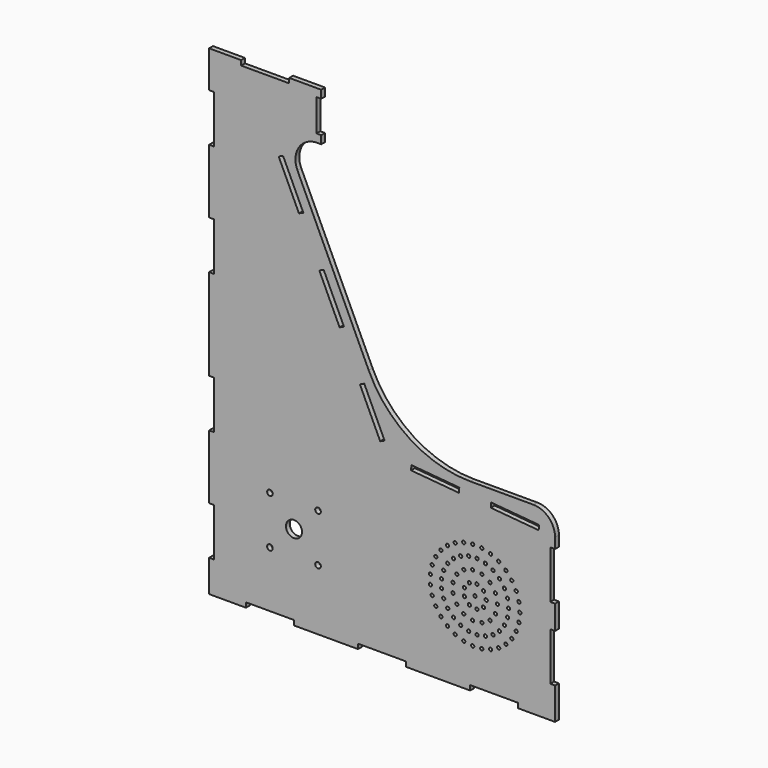
from build123d import *

# Parameters (mm, degrees)
F1_DEPTH = 3
F2_R     = 1.75
F2_R_2   = 5
F3_DEPTH = 3
F4_R     = 13.5
F5_R     = 70
F6_R     = 1
F7_DEPTH = 3


# Not quite as in the source:
# - a feature names something its author has since deleted; it is built from what else it names


with BuildPart() as f1:
    # F0 (on Front) → F1 (new body)
    with BuildSketch(Plane.XZ):
        Polygon((0, 20), (0, 0), (23, 0), (23, 3), (53, 3), (53, 0), (93, 0), (93, 3), (123, 3), (123, 0), (163, 0), (163, 3), (193, 3), (193, 0), (216, 0), (216, 20), (213, 20), (213, 50), (216, 50), (216, 65), (213, 65), (213, 95), (216, 95), (216, 115), (118.5, 115), (46.222312986, 270), (70, 270), (70, 275), (67, 275), (67, 295), (70, 295), (70, 300), (50, 300), (50, 297), (20, 297), (20, 300), (0, 300), (0, 277), (3, 277), (3, 247), (0, 247), (0, 207), (3, 207), (3, 177), (0, 177), (0, 120), (3, 120), (3, 90), (0, 90), (0, 50), (3, 50), (3, 20), align=None)
    extrude(amount=F1_DEPTH)

    # F2 (on face) → F3 (cut, through all)
    with BuildSketch(Plane.XZ.offset(3)):
        Polygon((156.2169022088, 109.3853277176), (126.331061266, 112), (126.0695940378, 109.0114159057), (155.9554349805, 106.3967436233), align=None)
        Polygon((206.0266371134, 105.0275405802), (176.1407961706, 107.6422128626), (175.8793289424, 104.6536287683), (205.7651698851, 102.0389564859), align=None)
        Polygon((84.1967806423, 174.3662818095), (71.51823279, 201.5555154206), (68.7993094289, 200.2876606354), (81.4778572811, 173.0984270243), align=None)
        Polygon((109.5538763467, 119.9878145873), (96.8753284945, 147.1770481984), (94.1564051334, 145.9091934132), (106.8349529856, 118.7199598021), align=None)
        Polygon((56.1207615767, 227.4768942465), (58.8396849378, 228.7447490317), (46.1611370856, 255.9339826428), (43.4422137245, 254.6661278576), align=None)
        with Locations((38, 68)):
            Circle(F2_R)
        with Locations((53, 53)):
            Circle(F2_R_2)
        with Locations((68, 68)):
            Circle(F2_R)
        with Locations((68, 38)):
            Circle(F2_R)
        with Locations((38, 38)):
            Circle(F2_R)
    extrude(amount=-F3_DEPTH, mode=Mode.SUBTRACT)

    # F4
    f4_edges = [f1.edges().sort_by_distance(p)[0] for p in [
        (216, -1.5, 115),
        (46.222313, -1.5, 270),
    ]]
    fillet(f4_edges, radius=F4_R)

    # F5
    f5_edges = [f1.edges().sort_by_distance(p)[0] for p in [
        (118.5, -1.5, 115),
    ]]
    fillet(f5_edges, radius=F5_R)

    # F6 (on face) → F7 (cut, through all)
    with BuildSketch(Plane.XZ.offset(3)):
        with Locations((166, 53)):
            Circle(F6_R)
        with Locations((173, 53)):
            Circle(F6_R)
        with Locations((180, 53)):
            Circle(F6_R)
        with Locations((187, 53)):
            Circle(F6_R)
        with Locations((171.3623111018, 57.4995132678)):
            Circle(F6_R)
        with Locations((167.2155372437, 59.8936542711)):
            Circle(F6_R)
        with Locations((162.5, 59.0621778265)):
            Circle(F6_R)
        with Locations((159.4221516545, 55.3941410033)):
            Circle(F6_R)
        with Locations((159.4221516545, 50.6058589967)):
            Circle(F6_R)
        with Locations((162.5, 46.9378221735)):
            Circle(F6_R)
        with Locations((167.2155372437, 46.1063457289)):
            Circle(F6_R)
        with Locations((178.789636407, 58.6943130031)):
            Circle(F6_R)
        with Locations((175.367828489, 63.4040275567)):
            Circle(F6_R)
        with Locations((170.3262379212, 66.3147912281)):
            Circle(F6_R)
        with Locations((164.5366015143, 66.9233065352)):
            Circle(F6_R)
        with Locations((159, 65.124355653)):
            Circle(F6_R)
        with Locations((154.6737620788, 61.2289935321)):
            Circle(F6_R)
        with Locations((152.3059335897, 55.9107636714)):
            Circle(F6_R)
        with Locations((152.3059335897, 50.0892363286)):
            Circle(F6_R)
        with Locations((154.6737620788, 44.7710064679)):
            Circle(F6_R)
        with Locations((159, 40.875644347)):
            Circle(F6_R)
        with Locations((164.5366015143, 39.0766934648)):
            Circle(F6_R)
        with Locations((170.3262379212, 39.6852087719)):
            Circle(F6_R)
        with Locations((175.367828489, 42.5959724433)):
            Circle(F6_R)
        with Locations((178.789636407, 47.3056869969)):
            Circle(F6_R)
        with Locations((186.3402463837, 58.2224876305)):
            Circle(F6_R)
        with Locations((184.4024402809, 63.1168271561)):
            Circle(F6_R)
        with Locations((181.3083411758, 67.3754892245)):
            Circle(F6_R)
        with Locations((177.2523626946, 70.7308864355)):
            Circle(F6_R)
        with Locations((172.4893568819, 72.9721868422)):
            Circle(F6_R)
        with Locations((167.3186009101, 73.958561297)):
            Circle(F6_R)
        with Locations((162.0649923937, 73.6280322653)):
            Circle(F6_R)
        with Locations((157.0586348771, 72.0013681018)):
            Circle(F6_R)
        with Locations((152.6140962153, 69.1807780983)):
            Circle(F6_R)
        with Locations((149.0106431181, 65.3434902981)):
            Circle(F6_R)
        with Locations((146.4746937963, 60.7306156064)):
            Circle(F6_R)
        with Locations((145.1655912724, 55.6319979049)):
            Circle(F6_R)
        with Locations((145.1655912724, 50.3680020951)):
            Circle(F6_R)
        with Locations((146.4746937963, 45.2693843936)):
            Circle(F6_R)
        with Locations((149.0106431181, 40.6565097019)):
            Circle(F6_R)
        with Locations((152.6140962153, 36.8192219017)):
            Circle(F6_R)
        with Locations((157.0586348771, 33.9986318982)):
            Circle(F6_R)
        with Locations((162.0649923937, 32.3719677347)):
            Circle(F6_R)
        with Locations((167.3186009101, 32.041438703)):
            Circle(F6_R)
        with Locations((172.4893568819, 33.0278131578)):
            Circle(F6_R)
        with Locations((177.2523626946, 35.2691135645)):
            Circle(F6_R)
        with Locations((181.3083411758, 38.6245107755)):
            Circle(F6_R)
        with Locations((184.4024402809, 42.8831728439)):
            Circle(F6_R)
        with Locations((186.3402463837, 47.7775123695)):
            Circle(F6_R)
        with Locations((194, 53)):
            Circle(F6_R)
        with Locations((193.4268383551, 58.6363585625)):
            Circle(F6_R)
        with Locations((191.7308187254, 64.0419639432)):
            Circle(F6_R)
        with Locations((188.9813763538, 68.9955100227)):
            Circle(F6_R)
        with Locations((185.2910737341, 73.2941980424)):
            Circle(F6_R)
        with Locations((180.8109922892, 76.7620392099)):
            Circle(F6_R)
        with Locations((175.7245470797, 79.2570597001)):
            Circle(F6_R)
        with Locations((170.2399777701, 80.6771130812)):
            Circle(F6_R)
        with Locations((164.5818232725, 80.9640622008)):
            Circle(F6_R)
        with Locations((158.9817290968, 80.1061593283)):
            Circle(F6_R)
        with Locations((153.6689637564, 78.138527108)):
            Circle(F6_R)
        with Locations((148.8610324887, 75.1417206343)):
            Circle(F6_R)
        with Locations((144.7547725646, 71.2384295162)):
            Circle(F6_R)
        with Locations((141.518294748, 66.5884549509)):
            Circle(F6_R)
        with Locations((139.2841008208, 61.3821674433)):
            Circle(F6_R)
        with Locations((138.143658945, 55.8327130156)):
            Circle(F6_R)
        with Locations((138.143658945, 50.1672869844)):
            Circle(F6_R)
        with Locations((139.2841008208, 44.6178325567)):
            Circle(F6_R)
        with Locations((141.518294748, 39.4115450491)):
            Circle(F6_R)
        with Locations((144.7547725646, 34.7615704838)):
            Circle(F6_R)
        with Locations((148.8610324887, 30.8582793657)):
            Circle(F6_R)
        with Locations((153.6689637564, 27.861472892)):
            Circle(F6_R)
        with Locations((158.9817290968, 25.8938406717)):
            Circle(F6_R)
        with Locations((164.5818232725, 25.0359377992)):
            Circle(F6_R)
        with Locations((170.2399777701, 25.3228869188)):
            Circle(F6_R)
        with Locations((175.7245470797, 26.7429402999)):
            Circle(F6_R)
        with Locations((180.8109922892, 29.2379607901)):
            Circle(F6_R)
        with Locations((185.2910737341, 32.7058019576)):
            Circle(F6_R)
        with Locations((188.9813763538, 37.0044899773)):
            Circle(F6_R)
        with Locations((191.7308187254, 41.9580360568)):
            Circle(F6_R)
        with Locations((193.4268383551, 47.3636414375)):
            Circle(F6_R)
        with Locations((171.3623111018, 48.5004867322)):
            Circle(F6_R)
    extrude(amount=-F7_DEPTH, mode=Mode.SUBTRACT)


solid = f1.part
